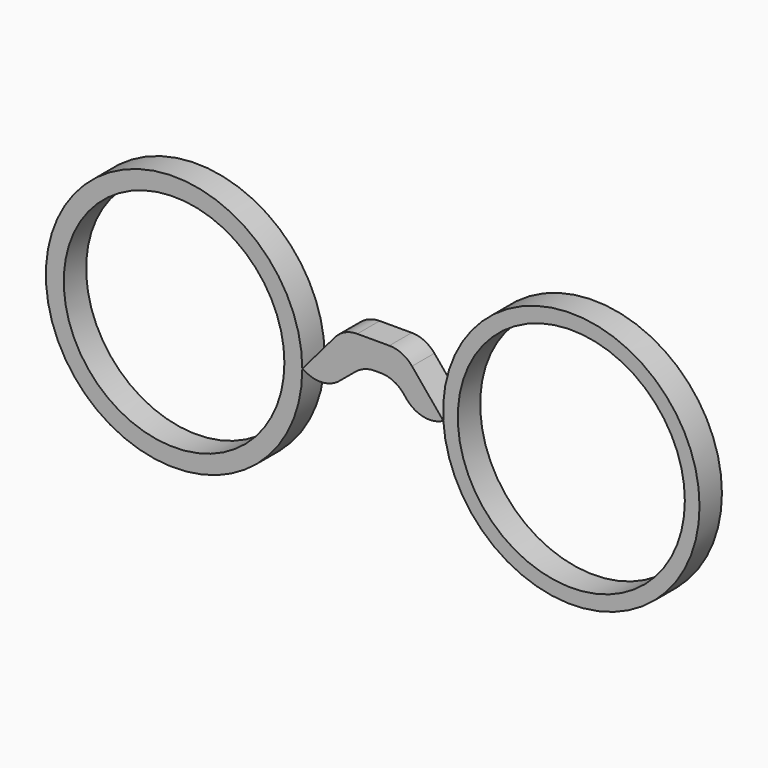
from build123d import *

# Parameters (mm, degrees)
F0_R         = 19.577599846
F1_DEPTH     = 4.826
F0_R_2       = 19.025309539
F2_T1_DEPTH  = 4.826
F2_T3_DEPTH  = 4.826
F2_T5_DEPTH  = 31.5234235451
F2_T7_DEPTH  = 16.7860194566
F2_T9_DEPTH  = 16.5531509264
F2_T11_DEPTH = 20.0834356368


# Not quite as in the source:
# - a fillet or chamfer that OpenCascade refuses, or shapes differently, is made with other operations: its cross-section is extruded or revolved along the edge and cut away or added


with BuildPart() as f1:
    # F0 (on Front) → F1 (new body)
    with BuildSketch(Plane.XZ):
        with BuildLine():
            ThreePointArc((13.6721328815, 2.8802125551), (36.442735195, -17.8102871686), (57.8485954466, 4.2891756172))
            ThreePointArc((57.8485954466, 4.2891756172), (35.0330556983, 26.3886384029), (13.6721328815, 2.8802125551))
        make_face()
        with Locations((35.7378954466, 4.2891756172)):
            Circle(F0_R, mode=Mode.SUBTRACT)
    extrude(amount=F1_DEPTH)


with BuildPart() as f1b:
    # F0 (on Front) → F1, piece 2 (new body)
    with BuildSketch(Plane.XZ):
        with BuildLine():
            ThreePointArc((-10.6526581482, 2.7790347432), (-10.6527160219, 2.8296237815), (-10.6528896426, 2.8802125551))
            ThreePointArc((-10.6528896426, 2.8802125551), (-54.8740002746, 2.7284457048), (-10.6526581482, 2.7790347432))
        make_face()
        with Locations((-32.7633581482, 2.7790347432)):
            Circle(F0_R_2, mode=Mode.SUBTRACT)
    extrude(amount=F1_DEPTH)


with BuildPart() as f1c:
    # F0 (on Front) → F1, piece 3 (new body)
    with BuildSketch(Plane.XZ):
        Polygon((10.7475112172, 0), (13.6721328815, 2.8802125551), (6.7447727473, 11.2624050619), (-3.5103600677, 11.2624050619), (-10.6528896426, 2.8802125551), (-7.0816248551, 1.0832078445), (-4.5412281389, 2.8802125551), (0, 6.6332548222), (5.2655391702, 6.6332548222), align=None)
    extrude(amount=F1_DEPTH)

    # F2: fillet of radius 5.08 on 6 edges, made by hand

    # F2_s2 → F2_t1 (join)
    with BuildSketch(Plane.XZ):
        with BuildLine():
            ThreePointArc((-1.4086830483, 5.4690660038), (0.1078865603, 6.3333552815), (1.8274910494, 6.6332548222))
            Line((1.8274910494, 6.6332548222), (0, 6.6332548222))
            Line((0, 6.6332548222), (-1.4086830483, 5.4690660038))
        make_face()
    extrude(amount=F2_T1_DEPTH)

    # F2_s4 → F2_t3 (join)
    with BuildSketch(Plane.XZ):
        with BuildLine():
            ThreePointArc((6.7893464605, 4.7894289199), (5.0376327333, 6.1492402669), (2.8735352789, 6.6332548222))
            Line((2.8735352789, 6.6332548222), (5.2655391702, 6.6332548222))
            Line((5.2655391702, 6.6332548222), (6.7893464605, 4.7894289199))
        make_face()
    extrude(amount=F2_T3_DEPTH)

    # F2_s6 → F2_t5 (cut)
    with BuildSketch(Plane.XZ.offset(-13.3487117726)):
        with BuildLine():
            ThreePointArc((13.6721328815, 2.8802125551), (10.2880191967, 2.3662176021), (7.3460344239, 4.1158295133))
            Line((7.3460344239, 4.1158295133), (10.7475112172, 0))
            Line((10.7475112172, 0), (13.6721328815, 2.8802125551))
        make_face()
    extrude(amount=F2_T5_DEPTH, mode=Mode.SUBTRACT)

    # F2_s8 → F2_t7 (cut)
    with BuildSketch(Plane.XZ.offset(-5.9800097283)):
        with BuildLine():
            ThreePointArc((8.2685800376, 9.4185791596), (6.5168663104, 10.7783905066), (4.352768856, 11.2624050619))
            Line((4.352768856, 11.2624050619), (6.7447727473, 11.2624050619))
            Line((6.7447727473, 11.2624050619), (8.2685800376, 9.4185791596))
        make_face()
    extrude(amount=F2_T7_DEPTH, mode=Mode.SUBTRACT)

    # F2_s10 → F2_t9 (cut)
    with BuildSketch(Plane.XZ.offset(-5.8635754632)):
        with BuildLine():
            ThreePointArc((-5.0315573811, 9.4771875716), (-3.2943552568, 10.7945572249), (-1.1649298824, 11.2624050619))
            Line((-1.1649298824, 11.2624050619), (-3.5103600677, 11.2624050619))
            Line((-3.5103600677, 11.2624050619), (-5.0315573811, 9.4771875716))
        make_face()
    extrude(amount=F2_T9_DEPTH, mode=Mode.SUBTRACT)

    # F2_s12 → F2_t11 (cut)
    with BuildSketch(Plane.XZ.offset(-7.6287178184)):
        with BuildLine():
            ThreePointArc((-4.5904071854, 2.84542469), (-7.1447926035, 1.9268884046), (-9.8074770052, 2.4548141088))
            Line((-9.8074770052, 2.4548141088), (-7.0816248551, 1.0832078445))
            Line((-7.0816248551, 1.0832078445), (-4.5904071854, 2.84542469))
        make_face()
    extrude(amount=F2_T11_DEPTH, mode=Mode.SUBTRACT)


solid = Compound([f1.part, f1b.part, f1c.part])
